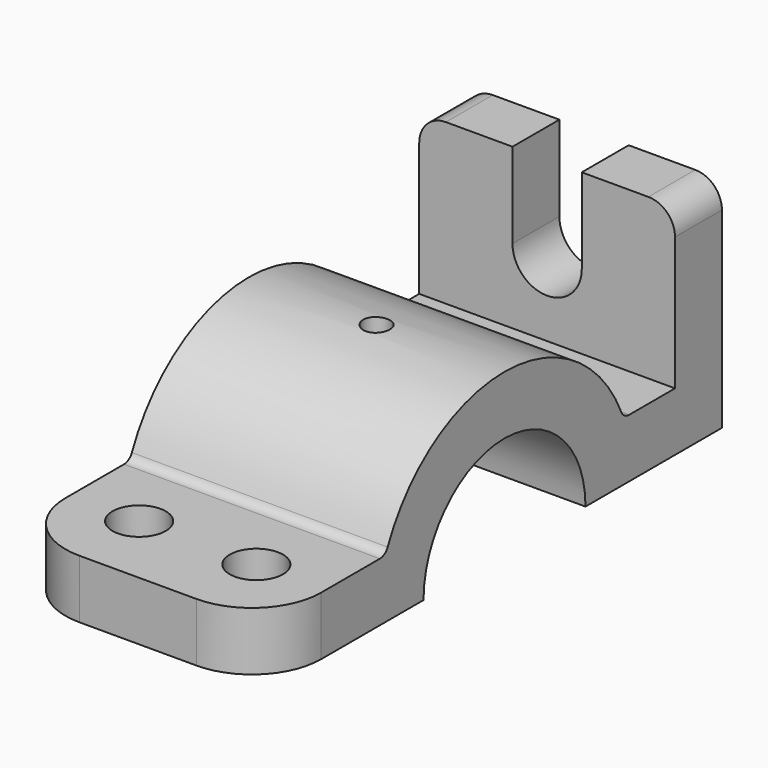
from build123d import *

# Parameters (mm, degrees)
F0_W     = 11
F0_H     = 30
F1_DEPTH = 24
F3_DEPTH = 11
F4_R     = 2.5
F4_R_2   = 5
F5_DEPTH = 41.001
F6_R     = 13
F7_R     = 5
F8_R     = 2


with BuildPart() as f1:
    # F0 (on Right) → F1 (new body, symmetric)
    with BuildSketch(Plane.YZ):
        with BuildLine():
            ThreePointArc((15.4919333848, 11), (18.1017503893, 5.7729223833), (19, 0))
            Line((19, 0), (30, 0))
            ThreePointArc((30, 0), (29.4730143031, 5.5983415304), (27.9105714739, 11))
            Line((27.9105714739, 11), (15.4919333848, 11))
        make_face()
        with BuildLine():
            ThreePointArc((-15.4919333848, 11), (0, 19), (15.4919333848, 11))
            Line((15.4919333848, 11), (27.9105714739, 11))
            ThreePointArc((27.9105714739, 11), (0, 30), (-27.9105714739, 11))
            Line((-27.9105714739, 11), (-15.4919333848, 11))
        make_face()
        with BuildLine():
            Line((-30, 0), (-19, 0))
            ThreePointArc((-19, 0), (-18.1017503893, 5.7729223833), (-15.4919333848, 11))
            Line((-15.4919333848, 11), (-27.9105714739, 11))
            ThreePointArc((-27.9105714739, 11), (-29.4730143031, 5.5983415304), (-30, 0))
        make_face()
        with BuildLine():
            ThreePointArc((27.9105714739, 11), (29.4730143031, 5.5983415304), (30, 0))
            Line((30, 0), (51, 0))
            Line((51, 0), (51, 11))
            Line((51, 11), (40, 11))
            Line((40, 11), (27.9105714739, 11))
        make_face()
        with BuildLine():
            Line((-56, 0), (-30, 0))
            ThreePointArc((-30, 0), (-29.4730143031, 5.5983415304), (-27.9105714739, 11))
            Line((-27.9105714739, 11), (-56, 11))
            Line((-56, 11), (-56, 0))
        make_face()
        with Locations((45.5, 26)):
            Rectangle(F0_W, F0_H)
    extrude(amount=F1_DEPTH, both=True)

    # F2 (on face) → F3 (cut, through all)
    with BuildSketch(Plane(origin=(0, 51, 0), x_dir=(-1, 0, 0), z_dir=(0, 1, 0))):
        with BuildLine():
            ThreePointArc((-6.5, 25), (0, 18.5), (6.5, 25))
            ThreePointArc((6.5, 25), (0, 31.5), (-6.5, 25))
        make_face()
        with BuildLine():
            ThreePointArc((-6.5, 25), (0, 31.5), (6.5, 25))
            Line((6.5, 25), (6.5, 41))
            Line((6.5, 41), (-6.5, 41))
            Line((-6.5, 41), (-6.5, 25))
        make_face()
    extrude(amount=-F3_DEPTH, mode=Mode.SUBTRACT)

    # F4 (on face) → F5 (cut, through all)
    with BuildSketch(Plane(origin=(0, 0, 0), x_dir=(1, 0, 0), z_dir=(0, 0, -1))):
        Circle(F4_R)
        with Locations((-11, 41.955285737)):
            Circle(F4_R_2)
        with Locations((11, 41.955285737)):
            Circle(F4_R_2)
    extrude(amount=-F5_DEPTH, mode=Mode.SUBTRACT)

    # F6
    f6_edges = [f1.edges().sort_by_distance(p)[0] for p in [
        (24, -56, 5.5),
        (-24, -56, 5.5),
    ]]
    fillet(f6_edges, radius=F6_R)

    # F7
    f7_edges = [f1.edges().sort_by_distance(p)[0] for p in [
        (24, 45.5, 41),
        (-24, 45.5, 41),
    ]]
    fillet(f7_edges, radius=F7_R)

    # F8
    f8_edges = [f1.edges().sort_by_distance(p)[0] for p in [
        (0, -27.910571, 11),
        (0, 27.910571, 11),
    ]]
    fillet(f8_edges, radius=F8_R)


solid = f1.part
